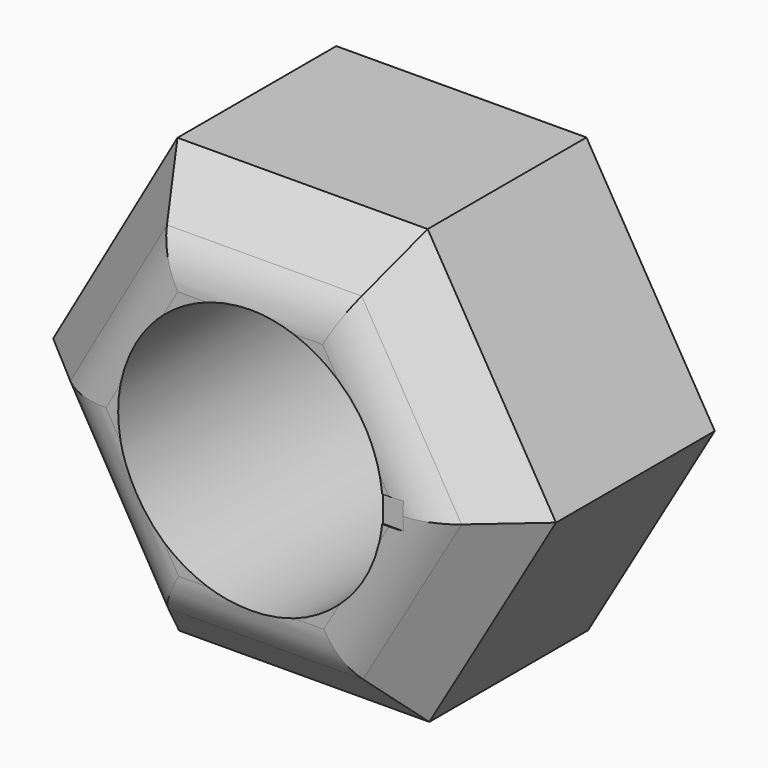
from build123d import *

# Parameters (mm, degrees)
F1_DEPTH     = 10
F2_SIZE      = 5
F3_T1_DEPTH  = 22.73867608
F3_T3_DEPTH  = 22.73867608
F3_T5_DEPTH  = 22.762654105
F3_T7_DEPTH  = 22.8342533194
F3_T9_DEPTH  = 22.7705922303
F3_T11_DEPTH = 22.7699440814
F0_W         = 1.5501256289
F0_H         = 2
F4_DEPTH     = 9.9305


# Not quite as in the source:
# - a fillet or chamfer that OpenCascade refuses, or shapes differently, is made with other operations: its cross-section is extruded or revolved along the edge and cut away or added


with BuildPart() as f1:
    # F0 (on Front) → F1 (new body, symmetric)
    with BuildSketch(Plane.XZ):
        Polygon((-9.3917044375, -16.4117172223), (9.5171118155, -16.3393132389), (19.091183747, 0.0319395585), (9.3917044375, 16.4117172223), (-9.5171118155, 16.3393132389), (-18.908816253, -0.0724039835), align=None)
        with BuildLine():
            ThreePointArc((9.9498743711, -1), (-10, 0), (9.9498743711, 1))
            Line((9.9498743711, 1), (11.5, 1))
            Line((11.5, 1), (11.5, -1))
            Line((11.5, -1), (9.9498743711, -1))
        make_face(mode=Mode.SUBTRACT)
    extrude(amount=F1_DEPTH, both=True)

    # F2
    f2_edges = [f1.edges().sort_by_distance(p)[0] for p in [
        (-14.212964, -10, 8.133455),
        (-14.15026, -10, -8.242061),
        (14.241444, -10, 8.221828),
        (0.062704, -10, -16.375515),
        (14.304148, -10, -8.153687),
        (-0.062704, -10, 16.375515),
    ]]
    chamfer(f2_edges, length=F2_SIZE)

    # F3: fillet of radius 4.6368466753 on 6 edges, made by hand

    # F3_s2 → F3_t1 (cut)
    with BuildSketch(Plane(origin=(5.6469256621, 0, 9.8678304624), x_dir=(0, 1, 0), z_dir=(-0.4966802502, 0, -0.8679335972))):
        with BuildLine():
            ThreePointArc((-10, -9.4549905003), (-9.6470410634, -11.2294349014), (-8.6418990521, -12.7337362278))
            Line((-8.6418990521, -12.7337362278), (-10, -11.3756352799))
            Line((-10, -11.3756352799), (-10, -9.4549905003))
        make_face()
    extrude(amount=F3_T1_DEPTH, mode=Mode.SUBTRACT)

    # F3_s4 → F3_t3 (cut)
    with BuildSketch(Plane(origin=(-5.7223290296, 0, 9.8242963078), x_dir=(0, 1, 0), z_dir=(0.5033124188, 0, -0.8641045128))):
        with BuildLine():
            ThreePointArc((-8.6418990521, -12.7337362278), (-9.6470410634, -11.2294349014), (-10, -9.4549905003))
            Line((-10, -9.4549905003), (-10, -11.3756352799))
            Line((-10, -11.3756352799), (-8.6418990521, -12.7337362278))
        make_face()
    extrude(amount=F3_T3_DEPTH, mode=Mode.SUBTRACT)

    # F3_s6 → F3_t5 (cut)
    with BuildSketch(Plane(origin=(11.393232541, 0, 0.0436259684), x_dir=(0, 1, 0), z_dir=(-0.999992669, 0, -0.0038290844))):
        with BuildLine():
            ThreePointArc((-10, -9.4549905003), (-9.6470410634, -11.2294349014), (-8.6418990521, -12.7337362278))
            Line((-8.6418990521, -12.7337362278), (-10, -11.3756352799))
            Line((-10, -11.3756352799), (-10, -9.4549905003))
        make_face()
    extrude(amount=F3_T5_DEPTH, mode=Mode.SUBTRACT)

    # F3_s8 → F3_t7 (cut)
    with BuildSketch(Plane(origin=(5.8897484246, 0, -9.9461802651), x_dir=(0, 1, 0), z_dir=(-0.5095280522, 0, 0.8604540453))):
        with BuildLine():
            ThreePointArc((-10, -9.5227156054), (-9.6470410634, -11.2971600064), (-8.6418990521, -12.8014613328))
            Line((-8.6418990521, -12.8014613328), (-10, -11.443360385))
            Line((-10, -11.443360385), (-10, -9.5227156054))
        make_face()
    extrude(amount=F3_T7_DEPTH, mode=Mode.SUBTRACT)

    # F3_s10 → F3_t9 (cut)
    with BuildSketch(Plane(origin=(-5.677308487, 0, -9.7079542659), x_dir=(0, 1, 0), z_dir=(0.5048217704, 0, 0.863223598))):
        with BuildLine():
            ThreePointArc((-8.6418990521, -12.8219374878), (-9.6470410634, -11.3176361614), (-10, -9.5431917603))
            Line((-10, -9.5431917603), (-10, -11.4638365399))
            Line((-10, -11.4638365399), (-8.6418990521, -12.8219374878))
        make_face()
    extrude(amount=F3_T9_DEPTH, mode=Mode.SUBTRACT)

    # F3_s12 → F3_t11 (cut)
    with BuildSketch(Plane(origin=(-11.3692546917, 0, -0.0435341545), x_dir=(0, 1, 0), z_dir=(0.999992669, 0, 0.0038290844))):
        with BuildLine():
            ThreePointArc((-8.6418990521, -12.7337362278), (-9.6470410634, -11.2294349014), (-10, -9.4549905003))
            Line((-10, -9.4549905003), (-10, -11.3756352799))
            Line((-10, -11.3756352799), (-8.6418990521, -12.7337362278))
        make_face()
    extrude(amount=F3_T11_DEPTH, mode=Mode.SUBTRACT)

    # F0 (on Front) → F4 (join)
    with BuildSketch(Plane.XZ):
        with Locations((10.7249371855, 0)):
            Rectangle(F0_W, F0_H)
    extrude(amount=F4_DEPTH)


solid = f1.part
